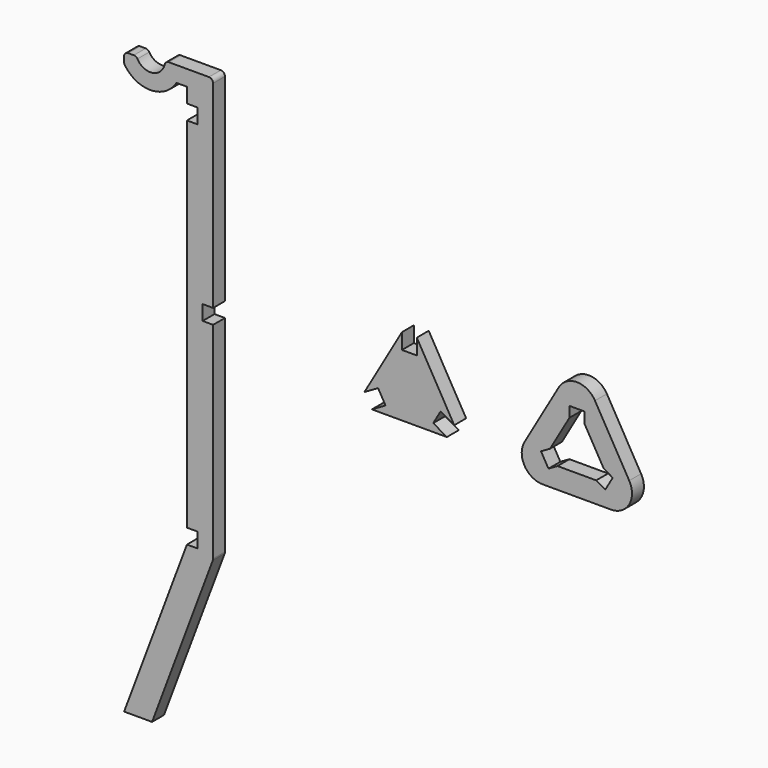
from build123d import *

# Parameters (mm, degrees)
F2_DEPTH = 18.034
F1_W     = 12.7
F1_H     = 19.05
F3_R     = 25.4
F4_R     = 5.08


# Not quite as in the source:
# - a variable given as a bare number and used for a length is read in inches; the dataset says mm whatever the document's units were


with BuildPart() as f2:
    # F1 (on Front) → F2 (new body)
    with BuildSketch(Plane.XZ):
        Polygon((457.2, 98.7234841871), (371.7029547439, -49.3617420935), (542.6970452561, -49.3617420935), align=None)
        Polygon((448.183, 32.3055820552), (448.183, 45.0055820552), (466.217, 45.0055820552), (466.217, 32.3055820552), (489.6859547439, -8.3438399617), (500.6844773719, -14.6938399617), (491.6674773719, -30.3117420935), (480.6689547439, -23.9617420935), (433.7310452561, -23.9617420935), (422.7325226281, -30.3117420935), (413.7155226281, -14.6938399617), (424.7140452561, -8.3438399617), align=None, mode=Mode.SUBTRACT)
    extrude(amount=F2_DEPTH)

    # F3
    f3_edges = [f2.edges().sort_by_distance(p)[0] for p in [
        (457.2, -9.017, 98.723484),
        (542.697045, -9.017, -49.361742),
        (371.702955, -9.017, -49.361742),
    ]]
    fillet(f3_edges, radius=F3_R)


with BuildPart() as f2b:
    # F1 (on Front) → F2, piece 2 (new body)
    with BuildSketch(Plane.XZ):
        Polygon((308.483, -21.0438399617), (263.017, 57.7055820552), (263.017, 38.6555820552), (244.983, 38.6555820552), (244.983, 57.7055820552), (199.517, -21.0438399617), (216.0147839421, -11.5188399617), (225.0317839421, -27.1367420935), (208.534, -36.6617420935), (299.466, -36.6617420935), (282.9682160579, -27.1367420935), (291.9852160579, -11.5188399617), align=None)
    extrude(amount=F2_DEPTH)


with BuildPart() as f2c:
    # F1 (on Front) → F2, piece 3 (new body)
    with BuildSketch(Plane.XZ):
        Polygon((15.875, 254), (-15.875, 254), (-15.875, 234.95), (-15.875, 216.9734554677), (-3.175, 216.9734554677), (-3.175, 198.9394554677), (-15.875, 198.9394554677), (-15.875, -235.966), (-3.175, -235.966), (-3.175, -254), (-15.875, -254), (-92.075, -457.2), (-58.1659851358, -457.2), (15.875, -259.7573729713), (15.875, -9.017), (3.175, -9.017), (3.175, 0), (3.175, 9.017), (15.875, 9.017), align=None)
        with Locations((-22.225, 244.475)):
            Rectangle(F1_W, F1_H)
        with BuildLine():
            Line((-28.575, 234.95), (-28.575, 254))
            Line((-28.575, 254), (-42.3484554677, 254))
            ThreePointArc((-42.3484554677, 254), (-57.0975584537, 236.315549927), (-77.1426589727, 247.65))
            Line((-77.1426589727, 247.65), (-92.075, 247.65))
            Line((-92.075, 247.65), (-92.075, 234.95))
            ThreePointArc((-92.075, 234.95), (-60.325, 216.9734554677), (-28.575, 234.95))
        make_face()
    extrude(amount=F2_DEPTH)

    # F4
    f4_edges = [f2c.edges().sort_by_distance(p)[0] for p in [
        (15.875, -9.017, -259.757373),
        (15.875, -9.017, 254),
        (-42.348455, -9.017, 254),
        (-77.142659, -9.017, 247.65),
        (-92.075, -9.017, 247.65),
        (-92.075, -9.017, 234.95),
    ]]
    fillet(f4_edges, radius=F4_R)


solid = Compound([f2.part, f2b.part, f2c.part])
